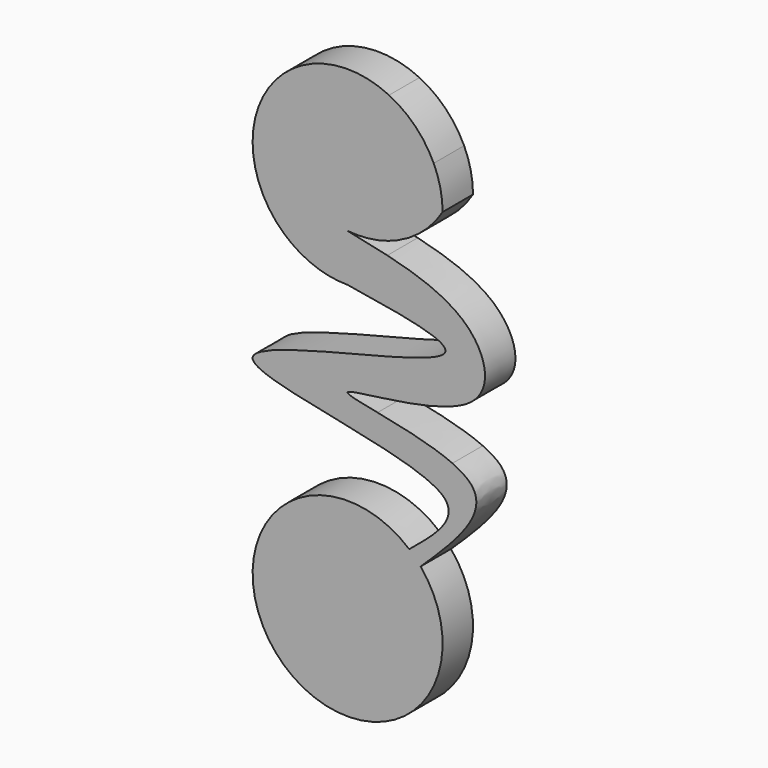
from build123d import *

# Parameters (mm, degrees)
F1_DEPTH = 3


# Not quite as in the source:
# - ends of sketch curves that miss each other by under 0.0002 mm in the source are joined


with BuildPart() as f1:
    # F0 (on Front) → F1 (new body)
    with BuildSketch(Plane.XZ):
        with BuildLine():
            add(Edge.make_bspline(
                [(7.5623651984, 10.2431356682), (8.8667882215, 8.9869659475), (6.8656342885, 7.3477267821), (4.8644803556, 5.7084876167)],
                knots=[0.8262576605, 0.8262576605, 0.8262576605, 0.8262576605, 1, 1, 1, 1], degree=3))
            ThreePointArc((4.8644803556, 5.7084876167), (-5.333479294, -5.2729497077), (5.7636359701, 4.7990103567))
            add(Edge.make_bspline(
                [(8.2732825601, 12.7880957686), (8.8398880918, 12.5318745493), (11.8721824839, 10.6993430744), (8.5602659443, 7.5003153724), (5.7636359701, 4.7990103567)],
                knots=[0.7696848931, 0.7696848931, 0.7696848931, 0.7696848931, 0.8055186102, 1, 1, 1, 1], degree=3))
            add(Edge.make_bspline(
                [(7.5623651984, 10.2431356682), (7.9881438125, 11.2069829018), (8.2451697716, 12.0771513969), (8.2732825613, 12.7880957689)],
                knots=[0.118501392, 0.118501392, 0.118501392, 0.118501392, 0.1544273329, 0.1544273329, 0.1544273329, 0.1544273329], degree=3))
        make_face()
        with BuildLine():
            add(Edge.make_bspline(
                [(-4.1962266618, 13.5761885948), (-0.2936458336, 12.6682093114), (5.9508638548, 11.7342957167), (7.5435064785, 10.2612967651), (7.5623651984, 10.2431356682)],
                knots=[0.6216232125, 0.6216232125, 0.6216232125, 0.6216232125, 0.8237457774, 0.8262576605, 0.8262576605, 0.8262576605, 0.8262576605], degree=3))
            add(Edge.make_bspline(
                [(7.5623651984, 10.2431356682), (7.9881438125, 11.2069829018), (8.2451697716, 12.0771513969), (8.2732825613, 12.7880957689)],
                knots=[0.118501392, 0.118501392, 0.118501392, 0.118501392, 0.1544273329, 0.1544273329, 0.1544273329, 0.1544273329], degree=3))
            add(Edge.make_bspline(
                [(2.3638817909, 14.3943168309), (4.1711140326, 14.0349387295), (6.6239413404, 13.5339342662), (8.2732825601, 12.7880957686)],
                knots=[0.6653759456, 0.6653759456, 0.6653759456, 0.6653759456, 0.7696848931, 0.7696848931, 0.7696848931, 0.7696848931], degree=3))
            add(Edge.make_bspline(
                [(2.3638817909, 14.3943168309), (0.1674386291, 14.0358440521), (-2.2670512459, 13.5498623866), (-4.1962266618, 13.5761885948)],
                knots=[0.2588323199, 0.2588323199, 0.2588323199, 0.2588323199, 0.3246194836, 0.3246194836, 0.3246194836, 0.3246194836], degree=3))
        make_face()
        with BuildLine():
            add(Edge.make_bspline(
                [(-7.2444975787, 14.5976251292), (-6.760519387, 14.2421388235), (-5.6315919935, 13.9101424686), (-4.1962266618, 13.5761885948)],
                knots=[0.5472827349, 0.5472827349, 0.5472827349, 0.5472827349, 0.6216232125, 0.6216232125, 0.6216232125, 0.6216232125], degree=3))
            add(Edge.make_bspline(
                [(2.3638817909, 14.3943168309), (0.1674386291, 14.0358440521), (-2.2670512459, 13.5498623866), (-4.1962266618, 13.5761885948)],
                knots=[0.2588323199, 0.2588323199, 0.2588323199, 0.2588323199, 0.3246194836, 0.3246194836, 0.3246194836, 0.3246194836], degree=3))
            add(Edge.make_bspline(
                [(3.1372160505, 25.5683519469), (5.8038062453, 24.9227331676), (10.5220974422, 23.2560876551), (12.1473944676, 15.6789716613), (-2.6978567307, 15.3734895471), (1.0303081424, 14.659505308), (2.3638817909, 14.3943168309)],
                knots=[0.0607215991, 0.0607215991, 0.0607215991, 0.0607215991, 0.2195316158, 0.3731691489, 0.5884053933, 0.6653759456, 0.6653759456, 0.6653759456, 0.6653759456], degree=3))
            add(Edge.make_bspline(
                [(3.1372160505, 25.5683519469), (2.1022005434, 24.0288162043), (1.0156251499, 22.8799200184), (-2.44874e-05, 22.5000654741)],
                knots=[0.7945343755, 0.7945343755, 0.7945343755, 0.7945343755, 0.844305066, 0.844305066, 0.844305066, 0.844305066], degree=3))
            add(Edge.make_bspline(
                [(-2.44874e-05, 22.5000654741), (4.3774352978, 21.8024255813), (14.9604012165, 20.1159571823), (-7.3551014619, 16.5428351503), (-7.5, 15)],
                knots=[0, 0, 0, 0, 0.2150812568, 0.5199842959, 0.5199842959, 0.5199842959, 0.5199842959], degree=3))
            add(Edge.make_bspline(
                [(-7.2444975787, 14.5976251292), (-7.3435869925, 14.7187439793), (-7.4291313398, 14.8525445582), (-7.5, 15)],
                knots=[0.3705375218, 0.3705375218, 0.3705375218, 0.3705375218, 0.378103182, 0.378103182, 0.378103182, 0.378103182], degree=3))
        make_face()
        with BuildLine():
            add(Edge.make_bspline(
                [(-7.5, 15), (-7.5129729895, 14.8618675908), (-7.4222183793, 14.7281626449), (-7.2444975787, 14.5976251292)],
                knots=[0.5199842959, 0.5199842959, 0.5199842959, 0.5199842959, 0.5472827349, 0.5472827349, 0.5472827349, 0.5472827349], degree=3))
            add(Edge.make_bspline(
                [(-7.2444975787, 14.5976251292), (-7.3435869925, 14.7187439793), (-7.4291313398, 14.8525445582), (-7.5, 15)],
                knots=[0.3705375218, 0.3705375218, 0.3705375218, 0.3705375218, 0.378103182, 0.378103182, 0.378103182, 0.378103182], degree=3))
        make_face()
        with BuildLine():
            ThreePointArc((-7.5, 30), (-6.8560792326, 26.9595760893), (-5.0348859849, 24.4412300714))
            ThreePointArc((-5.0348859849, 24.4412300714), (-3.7390178613, 23.498481298), (-2.2724478223, 22.8525542398))
            add(Edge.make_bspline(
                [(-2.2724478223, 22.8525542398), (-4.3888646939, 24.2552430986), (-6.1243013525, 28.2425079181), (-7.5, 30)],
                knots=[0.8835748226, 0.8835748226, 0.8835748226, 0.8835748226, 1, 1, 1, 1], degree=3))
        make_face()
        with BuildLine():
            add(Edge.make_bspline(
                [(3.1372160505, 25.5683519469), (2.1022005434, 24.0288162043), (1.0156251499, 22.8799200184), (-2.44874e-05, 22.5000654741)],
                knots=[0.7945343755, 0.7945343755, 0.7945343755, 0.7945343755, 0.844305066, 0.844305066, 0.844305066, 0.844305066], degree=3))
            add(Edge.make_bspline(
                [(0, 26.25), (1.0588176981, 26.0326033412), (2.1176353962, 25.8152066824), (3.1372160505, 25.5683519469)],
                knots=[0, 0, 0, 0, 0.0607215991, 0.0607215991, 0.0607215991, 0.0607215991], degree=3))
            ThreePointArc((0, 26.25), (2.0210303745, 26.313489261), (3.9594059157, 26.8890715071))
            add(Edge.make_bspline(
                [(6.8001792623, 33.1634730916), (6.0681213656, 31.0606340266), (5.0656540518, 28.7975749984), (3.9594059157, 26.8890715071)],
                knots=[0.7259897637, 0.7259897637, 0.7259897637, 0.7259897637, 0.7811375964, 0.7811375964, 0.7811375964, 0.7811375964], degree=3))
            ThreePointArc((6.8001792623, 33.1634730916), (5.3460226849, 35.2602320721), (3.2730609334, 36.7481161909))
            ThreePointArc((3.2730609334, 36.7481161909), (-3.9813341357, 36.3560190764), (-7.5, 30))
            add(Edge.make_bspline(
                [(-2.2724478223, 22.8525542398), (-4.3888646939, 24.2552430986), (-6.1243013525, 28.2425079181), (-7.5, 30)],
                knots=[0.8835748226, 0.8835748226, 0.8835748226, 0.8835748226, 1, 1, 1, 1], degree=3))
            ThreePointArc((-2.2724478223, 22.8525542398), (-1.1498166807, 22.5886626308), (-2.44874e-05, 22.5000654741))
        make_face()
        with BuildLine():
            add(Edge.make_bspline(
                [(6.8001792623, 33.1634730916), (6.0681213656, 31.0606340266), (5.0656540518, 28.7975749984), (3.9594059157, 26.8890715071)],
                knots=[0.7259897637, 0.7259897637, 0.7259897637, 0.7259897637, 0.7811375964, 0.7811375964, 0.7811375964, 0.7811375964], degree=3))
            ThreePointArc((3.9594059157, 26.8890715071), (5.9676703351, 28.1737015348), (7.5, 30))
            ThreePointArc((7.5, 30), (7.3229551571, 31.6199777056), (6.8001792623, 33.1634730916))
        make_face()
    extrude(amount=F1_DEPTH)


solid = f1.part
